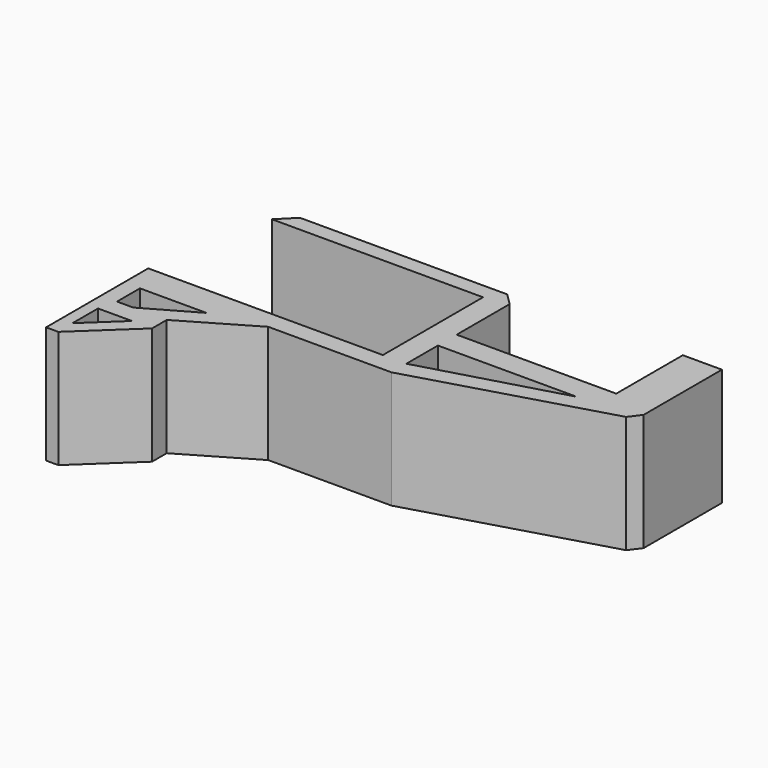
from build123d import *

# Parameters (mm, degrees)
F1_DEPTH    = 15
F2_T1_DEPTH = 22.7150489639
F2_T3_DEPTH = 20.8646002419
F3_SIZE     = 1.99999


# Not quite as in the source:
# - a fillet or chamfer that OpenCascade refuses, or shapes differently, is made with other operations: its cross-section is extruded or revolved along the edge and cut away or added
# - a fillet or chamfer is up to 0.001 mm smaller than in the source, because OpenCascade refuses the exact size


with BuildPart() as f1:
    # F0 (on Top) → F1 (new body)
    with BuildSketch(Plane.XY):
        Polygon((0, 16), (0, 0), (-30, 0), (-30, -2.3844742682), (-30, -16.3243375719), (-28.4316577017, -16.3243375719), (-21.5928480029, -9.9000008777), (-21.5928480029, -7.5513185002), (-12.7507485449, -2.3844742682), (3, -2.3844742682), (28.4, 5.0389636308), (28.4, 18.6757165939), (23.4, 18.6757165939), (23.4, 8.0389636308), (3, 8.0389636308), (3, 18), (-27, 18), (-27, 16), align=None)
        Polygon((-28.5007357597, -13.9756565914), (-28.5007357597, -10.7289487496), (-28.5007357597, -9.9000008777), (-24.1621347258, -9.9000008777), align=None, mode=Mode.SUBTRACT)
        Polygon((-27.9481057078, -3.890137421), (-19.4514021277, -3.890137421), (-25.8757378906, -7.5513185002), (-27.9481057078, -7.5513185002), align=None, mode=Mode.SUBTRACT)
        Polygon((3, 5.0389636308), (20.7205470651, 5.0389636308), (3, 0), align=None, mode=Mode.SUBTRACT)
    extrude(amount=F1_DEPTH)

    # F2: chamfer of 1.5 on 2 edges, made by hand

    # F2_s2 → F2_t1 (cut)
    with BuildSketch(Plane.XY.offset(-3.8575244819)):
        Polygon((1.5, 18), (3, 16.5), (3, 18), align=None)
    extrude(amount=F2_T1_DEPTH, mode=Mode.SUBTRACT)

    # F2_s4 → F2_t3 (cut)
    with BuildSketch(Plane.XY.offset(-2.932300121)):
        Polygon((28.4, 6.163321624), (27.3207889969, 4.7235519827), (28.4, 5.0389636308), align=None)
    extrude(amount=F2_T3_DEPTH, mode=Mode.SUBTRACT)

    # F3 (size 2 in the source; OpenCascade refuses exactly that, so slightly less here)
    f3_edges = [f1.edges().sort_by_distance(p)[0] for p in [
        (-27, 18, 7.5),
    ]]
    chamfer(f3_edges, length=F3_SIZE)


solid = f1.part
